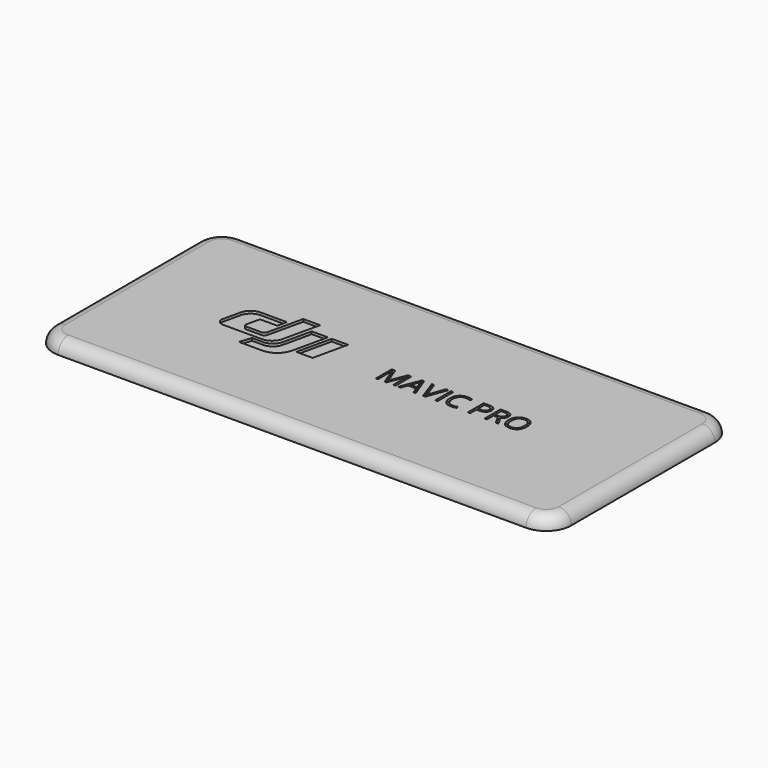
from build123d import *

# Parameters (mm, degrees)
F2_DEPTH     = 5
F3_R         = 4.99999
F1_TEXT_SIZE = 11.1039579173
F4_DEPTH     = 1


# Not quite as in the source:
# - a fillet or chamfer is up to 0.001 mm smaller than in the source, because OpenCascade refuses the exact size
# - Text() gives the source's letters only with a copy of the font that has no kerning and outlines rounded to 1/6400 em; it was checked with that copy


with BuildPart() as f2:
    # F0 (on Top) → F2 (new body)
    with BuildSketch(Plane.XY):
        with BuildLine():
            Line((93.3, 45.8), (-93.3, 45.8))
            ThreePointArc((-93.3, 45.8), (-100.3710678119, 42.8710678119), (-103.3, 35.8))
            Line((-103.3, 35.8), (-103.3, -35.8))
            ThreePointArc((-103.3, -35.8), (-100.3710678119, -42.8710678119), (-93.3, -45.8))
            Line((-93.3, -45.8), (93.3, -45.8))
            ThreePointArc((93.3, -45.8), (100.3710678119, -42.8710678119), (103.3, -35.8))
            Line((103.3, -35.8), (103.3, 35.8))
            ThreePointArc((103.3, 35.8), (100.3710678119, 42.8710678119), (93.3, 45.8))
        make_face()
    extrude(amount=-F2_DEPTH)

    # F3 (radius 5 in the source; OpenCascade refuses exactly that, so slightly less here)
    f3_edges = [f2.edges().sort_by_distance(p)[0] for p in [
        (103.3, 0, 0),
        (100.371068, 42.871068, 0),
        (0, 45.8, 0),
        (-100.371068, 42.871068, 0),
        (-103.3, 0, 0),
        (-100.371068, -42.871068, 0),
        (0, -45.8, 0),
        (100.371068, -42.871068, 0),
    ]]
    fillet(f3_edges, radius=F3_R)

    # F1 (on Top) → F4 (cut)
    with BuildSketch(Plane.XY):
        with BuildLine():
            Line((-36.1053960466, 13.3154064516), (-42.8327542772, 13.3154064516))
            Line((-42.8327542772, 13.3154064516), (-46.0113583328, -0.6546056617))
            ThreePointArc((-46.0113583328, -0.6546056617), (-46.5207475355, -1.4662094448), (-47.4251380852, -1.7828413984))
            Line((-47.4251380852, -1.7828413984), (-53.5277651889, -1.7828413984))
            ThreePointArc((-53.5277651889, -1.7828413984), (-54.2546478479, -1.4329448731), (-54.4345581584, -0.646549134))
            Line((-54.4345581584, -0.646549134), (-53.3793507787, 3.9911029982))
            ThreePointArc((-53.3793507787, 3.9911029982), (-53.0526304767, 4.5116625855), (-52.4725578093, 4.7147491192))
            Line((-52.4725578093, 4.7147491192), (-46.3379338884, 4.7147491192))
            Line((-46.3379338884, 4.7147491192), (-45.482161887, 8.4758797974))
            Line((-45.482161887, 8.4758797974), (-55.9513968165, 8.4758797974))
            ThreePointArc((-55.9513968165, 8.4758797974), (-59.0701703844, 7.3839805423), (-60.8267893381, 4.5851803703))
            Line((-60.8267893381, 4.5851803703), (-62.4010605499, -2.3337650266))
            ThreePointArc((-62.4010605499, -2.3337650266), (-61.92503295, -4.4145022292), (-60.0017623686, -5.3402991034))
            Line((-60.0017623686, -5.3402991034), (-44.420080815, -5.3402991034))
            ThreePointArc((-44.420080815, -5.3402991034), (-41.2389317758, -4.2265618632), (-39.4471804431, -1.3717856878))
            Line((-39.4471804431, -1.3717856878), (-36.1053960466, 13.3154064516))
        make_face()
        with BuildLine():
            Line((-29.0960520506, 8.4374961443), (-35.570547916, 8.4374961443))
            Line((-35.570547916, 8.4374961443), (-38.0946954232, -2.8365947523))
            ThreePointArc((-38.0946954232, -2.8365947523), (-39.8072515542, -5.5810030299), (-42.8595185073, -6.6525867845))
            Line((-42.8595185073, -6.6525867845), (-47.3061551221, -6.6525867845))
            Line((-47.3061551221, -6.6525867845), (-48.8149221495, -11.2701526103))
            Line((-48.8149221495, -11.2701526103), (-39.4923123752, -11.2701526103))
            ThreePointArc((-39.4923123752, -11.2701526103), (-34.8216252241, -9.6303771416), (-32.2010110907, -5.4307862549))
            Line((-32.2010110907, -5.4307862549), (-29.0960520506, 8.4374961443))
        make_face()
        Polygon((-30.6954588741, -5.3762982134), (-24.173093494, -5.3762982134), (-21.0803337395, 8.4374961443), (-27.6026991196, 8.4374961443), align=None)
        with Locations((-1.236253418, -3.8721226156)):
            Text('MAVIC PRO', F1_TEXT_SIZE, font='Open Sans', text_align=(TextAlign.LEFT, TextAlign.BOTTOM))
    extrude(amount=-F4_DEPTH, mode=Mode.SUBTRACT)


solid = f2.part
